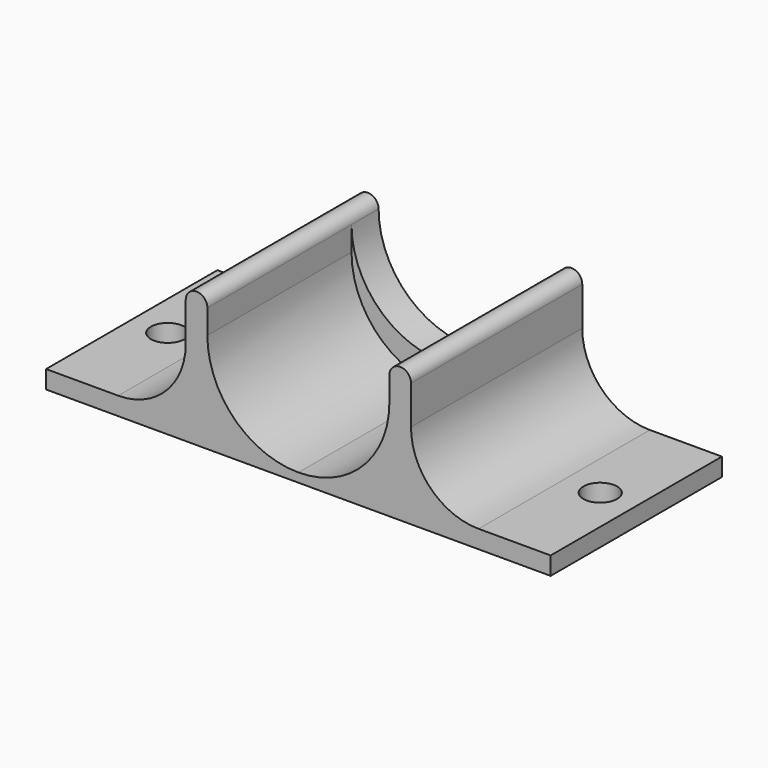
from build123d import *

# Parameters (mm, degrees)
F1_DEPTH = 25.4
F2_DEPTH = 4.7752
F4_D     = 4.7625


# Not quite as in the source:
# - a pattern or mirror of a feature is missing from the dataset's text; its kind, count and spacing are read off the source's solid


with BuildPart() as f1:
    # F0 (on Front) → F1 (new body)
    with BuildSketch(Plane.XZ):
        with BuildLine():
            Line((-35.56, 0), (0, 0))
            Line((0, 0), (35.56, 0))
            Line((35.56, 0), (35.56, 2.54))
            Line((35.56, 2.54), (25.4, 2.54))
            ThreePointArc((25.4, 2.54), (18.6648079092, 5.3298079092), (15.875, 12.065))
            Line((15.875, 12.065), (15.875, 17.526))
            ThreePointArc((15.875, 17.526), (14.351, 19.05), (12.827, 17.526))
            Line((12.827, 17.526), (12.827, 14.097))
            ThreePointArc((12.827, 14.097), (9.0700586823, 5.0269413177), (0, 1.27))
            ThreePointArc((0, 1.27), (-9.0700586823, 5.0269413177), (-12.827, 14.097))
            Line((-12.827, 14.097), (-12.827, 17.526))
            ThreePointArc((-12.827, 17.526), (-14.351, 19.05), (-15.875, 17.526))
            Line((-15.875, 17.526), (-15.875, 12.065))
            ThreePointArc((-15.875, 12.065), (-18.6648079092, 5.3298079092), (-25.4, 2.54))
            Line((-25.4, 2.54), (-35.56, 2.54))
            Line((-35.56, 2.54), (-35.56, 0))
        make_face()
    extrude(amount=F1_DEPTH)

    # F0 (on Front) → F2 (join)
    with BuildSketch(Plane.XZ):
        with BuildLine():
            Line((-35.56, 0), (0, 0))
            Line((0, 0), (35.56, 0))
            Line((35.56, 0), (35.56, 2.54))
            Line((35.56, 2.54), (25.4, 2.54))
            ThreePointArc((25.4, 2.54), (18.6648079092, 5.3298079092), (15.875, 12.065))
            Line((15.875, 12.065), (15.875, 17.526))
            ThreePointArc((15.875, 17.526), (14.351, 19.05), (12.827, 17.526))
            Line((12.827, 17.526), (12.827, 14.097))
            ThreePointArc((12.827, 14.097), (9.0700586823, 5.0269413177), (0, 1.27))
            ThreePointArc((0, 1.27), (-9.0700586823, 5.0269413177), (-12.827, 14.097))
            Line((-12.827, 14.097), (-12.827, 17.526))
            ThreePointArc((-12.827, 17.526), (-14.351, 19.05), (-15.875, 17.526))
            Line((-15.875, 17.526), (-15.875, 12.065))
            ThreePointArc((-15.875, 12.065), (-18.6648079092, 5.3298079092), (-25.4, 2.54))
            Line((-25.4, 2.54), (-35.56, 2.54))
            Line((-35.56, 2.54), (-35.56, 0))
        make_face()
        with BuildLine():
            ThreePointArc((0, 4.699), (-9.0700586823, 8.4559413177), (-12.827, 17.526))
            Line((-12.827, 17.526), (-12.827, 14.097))
            ThreePointArc((-12.827, 14.097), (-9.0700586823, 5.0269413177), (0, 1.27))
            ThreePointArc((0, 1.27), (9.0700586823, 5.0269413177), (12.827, 14.097))
            Line((12.827, 14.097), (12.827, 17.526))
            ThreePointArc((12.827, 17.526), (9.0700586823, 8.4559413177), (0, 4.699))
        make_face()
    extrude(amount=-F2_DEPTH)

    # F4 (through all)
    with Locations(Plane.XY.offset(2.54)):
        with Locations((-30.48, -10.3124)):
            f4 = Hole(F4_D / 2)

    # F4_copies: F4 across plane
    add(f4.mirror(Plane(origin=(0, 0, 0), x_dir=(0, 0, 1), z_dir=(1, 0, 0))), mode=Mode.SUBTRACT)


solid = f1.part
